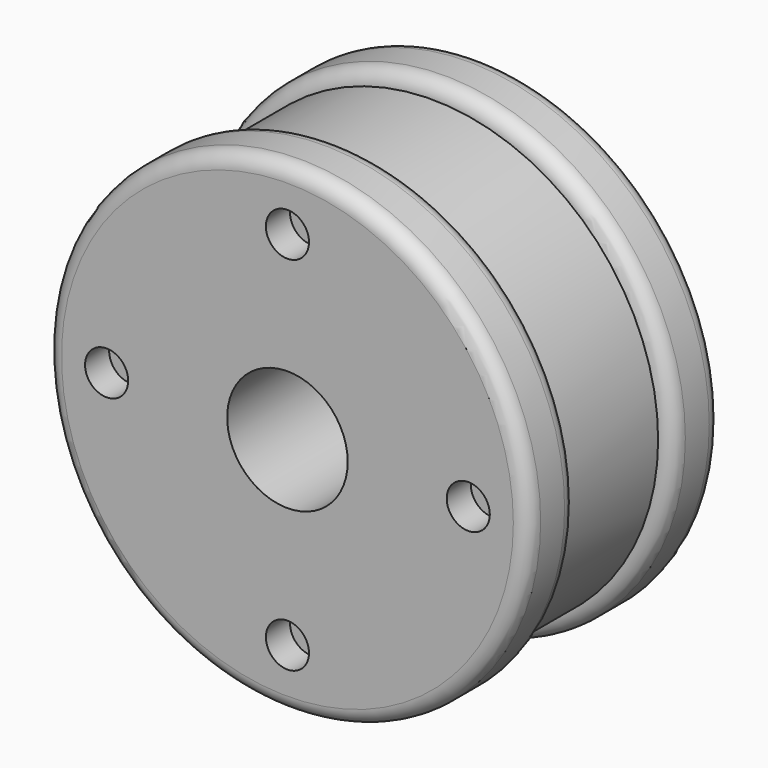
from build123d import *

# Parameters (mm, degrees)
F0_R         = 25.4
F1_DEPTH     = 6.35
F2_R         = 23.8125
F3_DEPTH     = 12.7
F4_R         = 25.4
F5_DEPTH     = 6.35
F6_S7_R      = 23.8125
F6_T8_DEPTH  = 40
F6_S13_R     = 23.8125
F6_T14_DEPTH = 40
F7_R         = 2.2698789725
F8_DEPTH     = 3.175
F9_R         = 6.35
F10_DEPTH    = 25.401


# Not quite as in the source:
# - a fillet or chamfer that OpenCascade refuses, or shapes differently, is made with other operations: its cross-section is extruded or revolved along the edge and cut away or added


with BuildPart() as f1:
    # F0 (on Front) → F1 (new body)
    with BuildSketch(Plane.XZ):
        Circle(F0_R)
    extrude(amount=F1_DEPTH)

    # F2 (on face) → F3 (join)
    with BuildSketch(Plane.XZ.offset(6.35)):
        Circle(F2_R)
    extrude(amount=F3_DEPTH)

    # F4 (on face) → F5 (join)
    with BuildSketch(Plane.XZ.offset(19.05)):
        Circle(F4_R)
    extrude(amount=F5_DEPTH)

    # F6: fillet of radius 1.6002 on 4 edges, made by hand

    # F6_s1 → F6_t2 (revolve, cut)
    with BuildSketch(Plane.XY):
        with BuildLine():
            ThreePointArc((25.4, -23.7998), (24.9313122713, -24.9313122713), (23.7998, -25.4))
            Line((23.7998, -25.4), (25.4, -25.4))
            Line((25.4, -25.4), (25.4, -23.7998))
        make_face()
    revolve(axis=Axis((0, -25.4, 0), (0, -1, 0)), mode=Mode.SUBTRACT)


with BuildPart() as f6_tool4:
    # F6_s5 → F6_t6 (revolve)
    with BuildSketch(Plane.XY):
        with BuildLine():
            ThreePointArc((25.4, -20.6502), (24.9313122713, -19.5186877287), (23.7998, -19.05))
            Line((23.7998, -19.05), (25.4, -19.05))
            Line((25.4, -19.05), (25.4, -20.6502))
        make_face()
    revolve(axis=Axis((0, -19.05, 0), (0, -1, 0)))

    # F6_s7 → F6_t8 (cut, symmetric)
    with BuildSketch(Plane.XZ.offset(19.9)):
        Circle(F6_S7_R)
    extrude(amount=F6_T8_DEPTH, both=True, mode=Mode.SUBTRACT)


with BuildPart() as f1_1:
    add(f1.part)

    # F6_t3: cut F6_tool4
    add(f6_tool4.part, mode=Mode.SUBTRACT)


with BuildPart() as f6_tool10:
    # F6_s11 → F6_t12 (revolve)
    with BuildSketch(Plane.XY):
        with BuildLine():
            ThreePointArc((23.7998, -6.35), (24.9313122713, -5.8813122713), (25.4, -4.7498))
            Line((25.4, -4.7498), (25.4, -6.35))
            Line((25.4, -6.35), (23.7998, -6.35))
        make_face()
    revolve(axis=Axis((0, -6.35, 0), (0, -1, 0)))

    # F6_s13 → F6_t14 (cut, symmetric)
    with BuildSketch(Plane.XZ.offset(5)):
        Circle(F6_S13_R)
    extrude(amount=F6_T14_DEPTH, both=True, mode=Mode.SUBTRACT)


with BuildPart() as f1_2:
    add(f1_1.part)

    # F6_t9: cut F6_tool10
    add(f6_tool10.part, mode=Mode.SUBTRACT)

    # F6_s15 → F6_t16 (revolve, cut)
    with BuildSketch(Plane.XY):
        with BuildLine():
            ThreePointArc((25.4, -1.6002), (24.9313122713, -0.4686877287), (23.7998, 0))
            Line((23.7998, 0), (25.4, 0))
            Line((25.4, 0), (25.4, -1.6002))
        make_face()
    revolve(axis=Axis((0, 0, 0), (0, -1, 0)), mode=Mode.SUBTRACT)

    # F7 (on face) → F8 (cut)
    with BuildSketch(Plane.XZ.offset(25.4)):
        with Locations((-19.05, 0)):
            Circle(F7_R)
        with Locations((0, -19.05)):
            Circle(F7_R)
        with Locations((19.05, 0)):
            Circle(F7_R)
        with Locations((0, 19.05)):
            Circle(F7_R)
    extrude(amount=-F8_DEPTH, mode=Mode.SUBTRACT)

    # F9 (on face) → F10 (cut, through all)
    with BuildSketch(Plane.XZ.offset(25.4)):
        Circle(F9_R)
    extrude(amount=-F10_DEPTH, mode=Mode.SUBTRACT)


solid = f1_2.part
